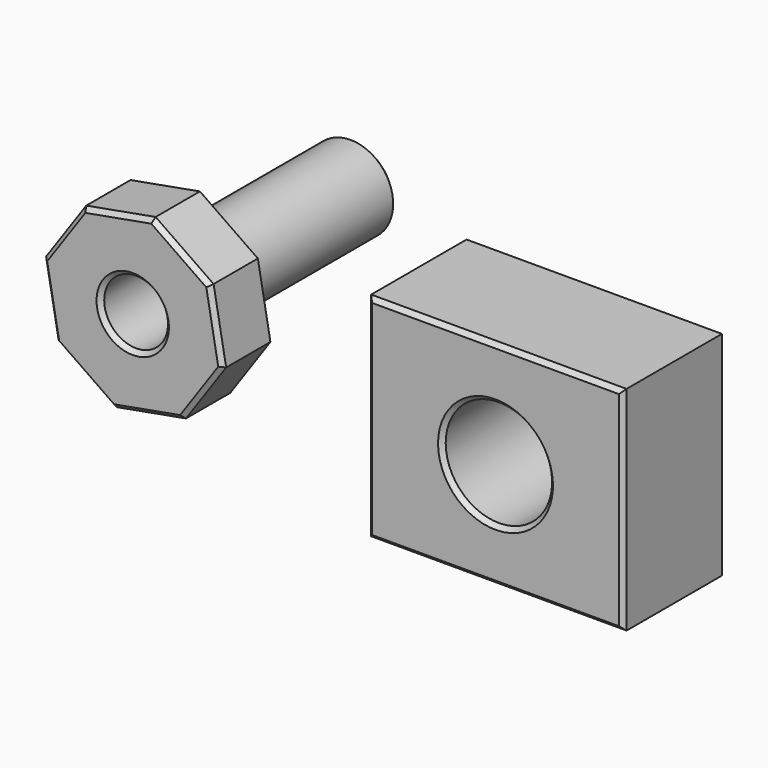
from build123d import *

# Parameters (mm, degrees)
F1_DEPTH = 30
F2_R     = 20
F3_DEPTH = 100
F5_D     = 30
F6_SIZE  = 2
F7_W     = 120
F7_H     = 100
F8_DEPTH = 60
F10_D    = 50
F11_SIZE = 2
F12_SIZE = 2


# Not quite as in the source:
# - a feature of the source that left no trace in its solid (it failed there, or was rolled back) is left out


with BuildPart() as f1:
    # F0 (on Front) → F1 (new body)
    with BuildSketch(Plane.XZ):
        Polygon((-23.4295373742, 36.4084245586), (-42.311828655, 9.1774591404), (-36.4084245586, -23.4295373742), (-9.1774591404, -42.311828655), (23.4295373742, -36.4084245586), (42.311828655, -9.1774591404), (36.4084245586, 23.4295373742), (9.1774591404, 42.311828655), align=None)
    extrude(amount=F1_DEPTH)

    # F2 (on face) → F3 (join)
    with BuildSketch(Plane(origin=(0, 0, 0), x_dir=(-1, 0, 0), z_dir=(0, 1, 0))):
        Circle(F2_R)
    extrude(amount=F3_DEPTH)

    # F5 (through all)
    with Locations(Plane.XZ.offset(30)):
        with Locations((0, 0)):
            Hole(F5_D / 2)

    # F6
    f6_edges = [f1.edges().sort_by_distance(p)[0] for p in [
        (20, 100, 0),
        (-7.126039, 0, 39.360127),
        (-7.126039, -30, 39.360127),
        (22.792942, 0, 32.870683),
        (22.792942, -30, 32.870683),
        (-32.870683, 0, 22.792942),
        (-32.870683, -30, 22.792942),
        (39.360127, 0, 7.126039),
        (-39.360127, 0, -7.126039),
        (32.870683, 0, -22.792942),
        (-22.792942, 0, -32.870683),
        (7.126039, 0, -39.360127),
        (20, 0, 0),
        (39.360127, -30, 7.126039),
        (-39.360127, -30, -7.126039),
        (32.870683, -30, -22.792942),
        (-22.792942, -30, -32.870683),
        (7.126039, -30, -39.360127),
        (-15, -30, 0),
        (-15, 100, 0),
    ]]
    chamfer(f6_edges, length=F6_SIZE)


with BuildPart() as f8:
    # F7 (on face) → F8 (new body)
    with BuildSketch(Plane.XZ.offset(30)):
        with Locations((218.4767627038, 33.1561379135)):
            Rectangle(F7_W, F7_H)
    extrude(amount=F8_DEPTH)

    # F10 (through all)
    with Locations(Plane.XZ.offset(90)):
        with Locations((218.4767627038, 33.1561379135)):
            Hole(F10_D / 2)

    # F11
    f11_edges = [f8.edges().sort_by_distance(p)[0] for p in [
        (218.476763, -90, 83.156138),
        (278.476763, -90, 33.156138),
        (158.476763, -90, 33.156138),
        (218.476763, -90, -16.843862),
        (193.476763, -90, 33.156138),
    ]]
    chamfer(f11_edges, length=F11_SIZE)

    # F12
    f12_edges = [f8.edges().sort_by_distance(p)[0] for p in [
        (218.476763, -30, 83.156138),
        (278.476763, -30, 33.156138),
        (158.476763, -30, 33.156138),
        (218.476763, -30, -16.843862),
        (193.476763, -30, 33.156138),
    ]]
    chamfer(f12_edges, length=F12_SIZE)


solid = Compound([f1.part, f8.part])
